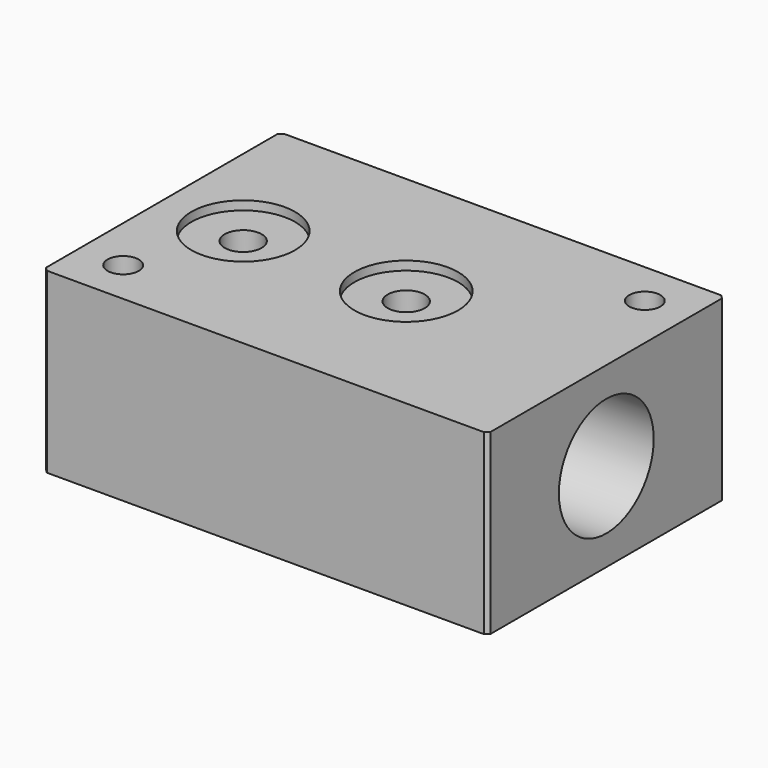
from build123d import *

# Parameters (mm, degrees)
F0_W      = 30
F0_H      = 20
F1_DEPTH  = 12
F2_R      = 4
F3_DEPTH  = 30
F4_R      = 1.25
F5_DEPTH  = 25
F4_R_2    = 1.05
F8_DEPTH  = 25
F9_SIZE   = 0.25
F4_R_3    = 3.5
F4_R_4    = 2.5
F10_DEPTH = 0.6


with BuildPart() as f1:
    # F0 (on Top) → F1 (new body)
    with BuildSketch(Plane.XY):
        with Locations((15, -10)):
            Rectangle(F0_W, F0_H)
    extrude(amount=F1_DEPTH)

    # F2 (on face) → F3 (cut)
    with BuildSketch(Plane(origin=(0, 0, 0), x_dir=(0, -1, 0), z_dir=(-1, 0, 0))):
        with Locations((10, 6)):
            Circle(F2_R)
    extrude(amount=-F3_DEPTH, mode=Mode.SUBTRACT)

    # F4 (on face) → F5 (cut)
    with BuildSketch(Plane.XY.offset(12)):
        with Locations((5.5, -10)):
            Circle(F4_R)
        with Locations((16.5, -10)):
            Circle(F4_R)
    extrude(amount=-F5_DEPTH, mode=Mode.SUBTRACT)

    # F4 (on face) → F8 (cut)
    with BuildSketch(Plane.XY.offset(12)):
        with Locations((3, -17)):
            Circle(F4_R_2)
        with Locations((27, -3)):
            Circle(F4_R_2)
    extrude(amount=-F8_DEPTH, mode=Mode.SUBTRACT)

    # F9
    f9_edges = [f1.edges().sort_by_distance(p)[0] for p in [
        (0, -6, 6),
        (0, 0, 6),
        (0, -20, 6),
        (30, 0, 6),
        (30, -20, 6),
    ]]
    chamfer(f9_edges, length=F9_SIZE)

    # F4 (on face) → F10 (cut)
    with BuildSketch(Plane.XY.offset(12)):
        with Locations((5.5, -10)):
            Circle(F4_R_3)
        with Locations((5.5, -10)):
            Circle(F4_R_4, mode=Mode.SUBTRACT)
        with Locations((16.5, -10)):
            Circle(F4_R_3)
        with Locations((16.5, -10)):
            Circle(F4_R_4, mode=Mode.SUBTRACT)
        with Locations((16.5, -10)):
            Circle(F4_R_4)
        with Locations((16.5, -10)):
            Circle(F4_R, mode=Mode.SUBTRACT)
        with Locations((5.5, -10)):
            Circle(F4_R_4)
        with Locations((5.5, -10)):
            Circle(F4_R, mode=Mode.SUBTRACT)
    extrude(amount=-F10_DEPTH, mode=Mode.SUBTRACT)


solid = f1.part
